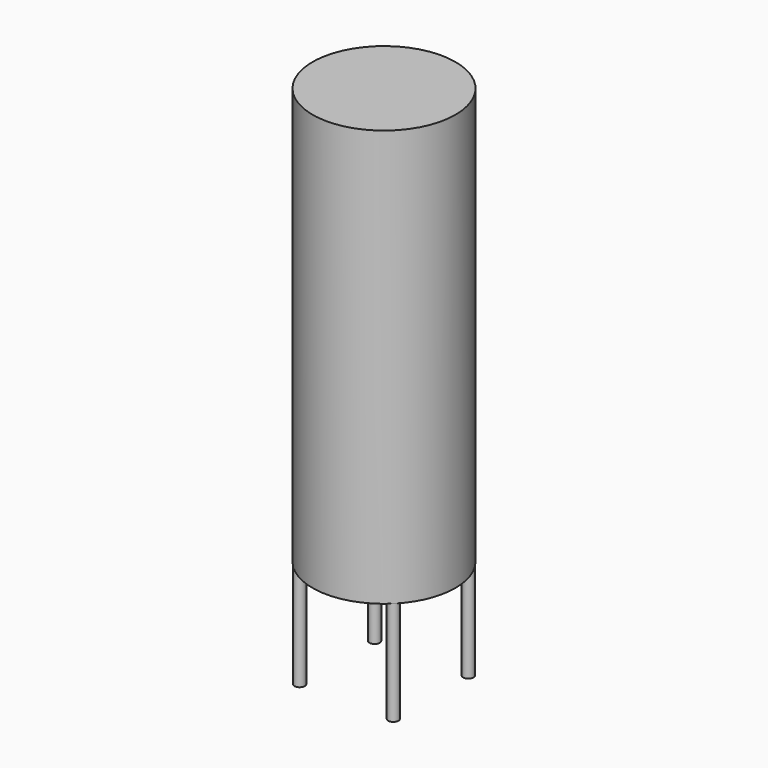
from build123d import *

# Parameters (mm, degrees)
F0_R     = 2.5
F1_DEPTH = 50
F2_R     = 34.3198051534
F3_DEPTH = 200


# Not quite as in the source:
# - a feature of the source that left no trace in its solid (it failed there, or was rolled back) is left out


with BuildPart() as f1:
    # F0 (on Top) → F1 (new body)
    with BuildSketch(Plane.XY):
        with Locations((0, 45)):
            Circle(F0_R)
    extrude(amount=F1_DEPTH)



with BuildPart() as f1b:
    # F0 (on Top) → F1, piece 2 (new body)
    with BuildSketch(Plane.XY):
        with Locations((45, 45)):
            Circle(F0_R)
    extrude(amount=F1_DEPTH)


with BuildPart() as f1c:
    # F0 (on Top) → F1, piece 3 (new body)
    with BuildSketch(Plane.XY):
        Circle(F0_R)
    extrude(amount=F1_DEPTH)


with BuildPart() as f1d:
    # F0 (on Top) → F1, piece 4 (new body)
    with BuildSketch(Plane.XY):
        with Locations((45, 0)):
            Circle(F0_R)
    extrude(amount=F1_DEPTH)


with BuildPart() as f1_1:
    add(f1.part)

    add(f1b.part)  # F3 merges F1b

    add(f1c.part)  # F3 merges F1c

    add(f1d.part)  # F3 merges F1d
    # F2 (on face) → F3 (join)
    with BuildSketch(Plane.XY.offset(50)):
        with Locations((22.5, 22.5)):
            Circle(F2_R)
    extrude(amount=F3_DEPTH)


solid = f1_1.part
